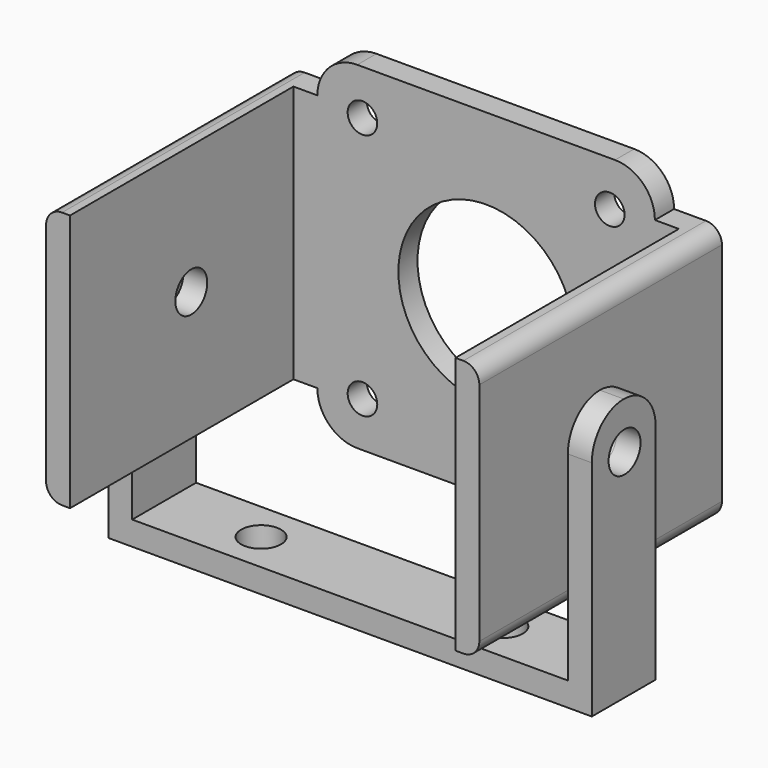
from build123d import *

# Parameters (mm, degrees)
F0_R           = 1.855
F1_DEPTH       = 3
F2_R           = 5
F3_W           = 3
F3_H           = 32.3
F4_DEPTH       = 3
F5_DEPTH       = 38
F6_R           = 2
F8_R           = 11
F9_DEPTH       = 3.001
F10_W          = 10
F10_H          = 3
F11_DEPTH      = 3
F12_R          = 4.99999
F13_DEPTH      = 54.6
F14_W          = 10
F14_H          = 30
F14_H_2        = 3
F15_DEPTH      = 3
F16_DEPTH      = 57.601
F16_DEPTH_BACK = 3.001
F17_R          = 4.99999
F19_DEPTH      = 25


# Not quite as in the source:
# - a fillet or chamfer is up to 0.001 mm smaller than in the source, because OpenCascade refuses the exact size


with BuildPart() as f1:
    # F0 (on Front) → F1 (new body)
    with BuildSketch(Plane.XZ):
        Polygon((29.887046665, 15.2593358934), (-12.412953335, 15.2593358934), (-12.412953335, 9.6093358934), (-12.412953335, -27.0406641066), (29.887046665, -27.0406641066), align=None)
        with Locations((-6.762953335, -21.3906641066)):
            Circle(F0_R, mode=Mode.SUBTRACT)
        with Locations((24.237046665, -21.3906641066)):
            Circle(F0_R, mode=Mode.SUBTRACT)
        with BuildLine():
            ThreePointArc((-4.907953335, 9.6093358934), (-6.762953335, 7.7543358934), (-8.617953335, 9.6093358934))
            ThreePointArc((-8.617953335, 9.6093358934), (-6.762953335, 11.4643358934), (-4.907953335, 9.6093358934))
        make_face(mode=Mode.SUBTRACT)
        with Locations((24.237046665, 9.6093358934)):
            Circle(F0_R, mode=Mode.SUBTRACT)
    extrude(amount=F1_DEPTH)

    # F2
    f2_edges = [f1.edges().sort_by_distance(p)[0] for p in [
        (29.887047, -1.5, 15.259336),
        (29.887047, -1.5, -27.040664),
        (-12.412953, -1.5, 15.259336),
        (-12.412953, -1.5, -27.040664),
    ]]
    fillet(f2_edges, radius=F2_R)

    # F3 (on face) → F4 (join)
    with BuildSketch(Plane(origin=(0, 0, 0), x_dir=(-1, 0, 0), z_dir=(0, 1, 0))):
        with Locations((13.912953335, -5.8906641066)):
            Rectangle(F3_W, F3_H)
        with Locations((-31.387046665, -5.8906641066)):
            Rectangle(F3_W, F3_H)
    extrude(amount=-F4_DEPTH)

    # F3 (on face) → F5 (join)
    with BuildSketch(Plane(origin=(0, 0, 0), x_dir=(-1, 0, 0), z_dir=(0, 1, 0))):
        with Locations((16.912953335, -5.8906641066)):
            Rectangle(F3_W, F3_H)
        with Locations((-34.387046665, -5.8906641066)):
            Rectangle(F3_W, F3_H)
    extrude(amount=-F5_DEPTH)

    # F6
    f6_edges = [f1.edges().sort_by_distance(p)[0] for p in [
        (35.887047, -19, -22.040664),
        (-18.412953, -19, -22.040664),
        (-18.412953, -19, 10.259336),
        (35.887047, -19, 10.259336),
    ]]
    fillet(f6_edges, radius=F6_R)

    # F8 (on face) → F9 (cut, through all)
    with BuildSketch(Plane.XZ.offset(3)):
        with Locations((8.737046665, -5.8906641066)):
            Circle(F8_R)
    extrude(amount=-F9_DEPTH, mode=Mode.SUBTRACT)


with BuildPart() as f11:
    # F10 (on face) → F11 (new body)
    with BuildSketch(Plane.YZ.offset(35.887046665)):
        Polygon((-14.1340063512, 0), (-19, 0), (-24.1340063512, 0), (-24.1340063512, -30), (-14.1340063512, -30), align=None)
        with Locations((-19.1340063512, -31.5)):
            Rectangle(F10_W, F10_H)
    extrude(amount=F11_DEPTH)

    # F12 (radius 5 in the source; OpenCascade refuses exactly that, so slightly less here)
    f12_edges = [f11.edges().sort_by_distance(p)[0] for p in [
        (37.387047, -24.134006, 0),
        (37.387047, -14.134006, 0),
    ]]
    fillet(f12_edges, radius=F12_R)

    # F10 (on face) → F13 (join)
    with BuildSketch(Plane.YZ.offset(35.887046665)):
        with Locations((-19.1340063512, -31.5)):
            Rectangle(F10_W, F10_H)
    extrude(amount=-F13_DEPTH)

    # F14 (on face) → F15 (join)
    with BuildSketch(Plane(origin=(-18.712953335, 0, 0), x_dir=(0, -1, 0), z_dir=(-1, 0, 0))):
        with Locations((19.1340063512, -15)):
            Rectangle(F14_W, F14_H)
        with Locations((19.1340063512, -31.5)):
            Rectangle(F14_W, F14_H_2)
    extrude(amount=F15_DEPTH)


with BuildPart() as f16_tool:
    # F7 (on face) → F16 (new body, two sides)
    with BuildSketch(Plane.YZ.offset(35.887046665)) as f16_sk:
        with BuildLine():
            Line((-21.5, -5.8906641066), (-19, -5.8906641066))
            Line((-19, -5.8906641066), (-16.5, -5.8906641066))
            ThreePointArc((-16.5, -5.8906641066), (-19, -3.3906641066), (-21.5, -5.8906641066))
        make_face()
        with BuildLine():
            Line((-16.5, -5.8906641066), (-19, -5.8906641066))
            Line((-19, -5.8906641066), (-21.5, -5.8906641066))
            ThreePointArc((-21.5, -5.8906641066), (-19, -8.3906641066), (-16.5, -5.8906641066))
        make_face()
    extrude(amount=-F16_DEPTH)
    extrude(f16_sk.sketch, amount=F16_DEPTH_BACK)


with BuildPart() as f1_1:
    add(f1.part)

    # F16: cut by f16_tool
    add(f16_tool.part, mode=Mode.SUBTRACT)


with BuildPart() as f11_1:
    add(f11.part)

    # F16: cut by f16_tool
    add(f16_tool.part, mode=Mode.SUBTRACT)

    # F17 (radius 5 in the source; OpenCascade refuses exactly that, so slightly less here)
    f17_edges = [f11_1.edges().sort_by_distance(p)[0] for p in [
        (-20.212953, -14.134006, 0),
        (-20.212953, -24.134006, 0),
    ]]
    fillet(f17_edges, radius=F17_R)

    # F18 (on face) → F19 (cut)
    with BuildSketch(Plane(origin=(0, 0, -33), x_dir=(1, 0, 0), z_dir=(0, 0, -1))):
        with BuildLine():
            Line((-9.062953335, 19.1340063512), (-6.562953335, 19.1340063512))
            Line((-6.562953335, 19.1340063512), (-4.062953335, 19.1340063512))
            ThreePointArc((-4.062953335, 19.1340063512), (-6.562953335, 21.6340063512), (-9.062953335, 19.1340063512))
        make_face()
        with BuildLine():
            Line((-4.062953335, 19.1340063512), (-6.562953335, 19.1340063512))
            Line((-6.562953335, 19.1340063512), (-9.062953335, 19.1340063512))
            ThreePointArc((-9.062953335, 19.1340063512), (-6.562953335, 16.6340063512), (-4.062953335, 19.1340063512))
        make_face()
        with BuildLine():
            ThreePointArc((26.237046665, 19.1340063512), (23.737046665, 21.6340063512), (21.237046665, 19.1340063512))
            Line((21.237046665, 19.1340063512), (23.737046665, 19.1340063512))
            Line((23.737046665, 19.1340063512), (26.237046665, 19.1340063512))
        make_face()
        with BuildLine():
            Line((23.737046665, 19.1340063512), (21.237046665, 19.1340063512))
            ThreePointArc((21.237046665, 19.1340063512), (23.737046665, 16.6340063512), (26.237046665, 19.1340063512))
            Line((26.237046665, 19.1340063512), (23.737046665, 19.1340063512))
        make_face()
    extrude(amount=-F19_DEPTH, mode=Mode.SUBTRACT)


solid = Compound([f1_1.part, f11_1.part])
